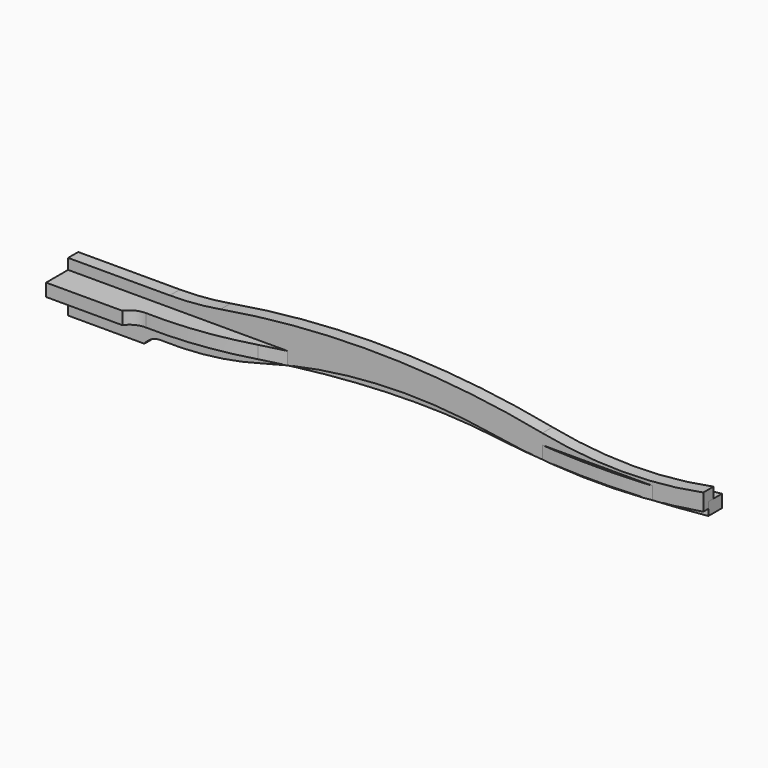
from build123d import *

# Parameters (mm, degrees)
F1_DEPTH = 7.5
F3_ANGLE = 90


# Not quite as in the source:
# - a feature of the source that left no trace in its solid (it failed there, or was rolled back) is left out


with BuildPart() as f1:
    # F0 (on Front) → F1 (new body, symmetric)
    with BuildSketch(Plane.XZ):
        with BuildLine():
            Line((-255, 20), (-315, 20))
            Line((-315, 20), (-375, 20))
            Line((-375, 20), (-375, -40))
            Line((-375, -40), (-285, -40))
            ThreePointArc((-285, -40), (-276.2591025809, -32.4817948381), (-265, -30))
            ThreePointArc((-265, -30), (-204.4210160851, -27.1318713195), (-145, -15))
            ThreePointArc((-145, -15), (-10.8395299917, 7.61153985), (125, 0))
            ThreePointArc((125, 0), (250, -10.4900271125), (375, 0))
            Line((375, 0), (375, 20))
            ThreePointArc((375, 20), (280, 10.6761525183), (185, 20))
            ThreePointArc((185, 20), (-4.7678400969, 39.906354128), (-195, 25.0799787))
            ThreePointArc((-195, 25.0799787), (-224.8926662439, 21.2722625064), (-255, 20))
        make_face()
    extrude(amount=F1_DEPTH, both=True)


with BuildPart() as f3_1:
    # F3: copy of F1
    add(f1.part.rotate(Axis((-189.5504295826, 0, 0), (-1, 0, 0)), F3_ANGLE))


solid = Compound([f1.part, f3_1.part])
